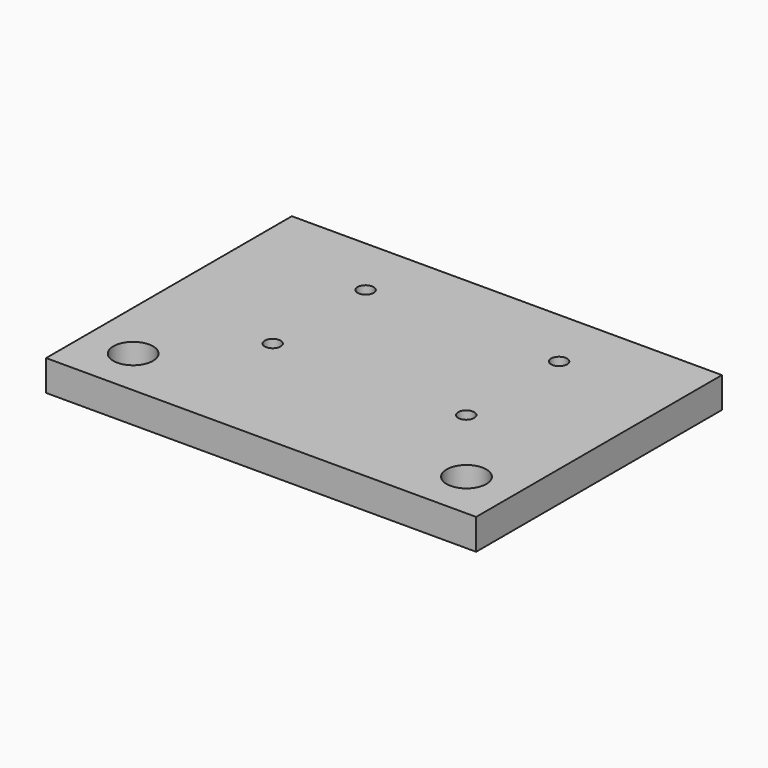
from build123d import *

# Parameters (mm, degrees)
F0_W           = 88.9
F0_H           = 63.5
F1_DEPTH       = 6.35
F2_D           = 8.2042
F3_D           = 3.3
F3_CBORE_D     = 8.25
F3_CBORE_DEPTH = 4


# Not quite as in the source:
# - a feature names something its author has since deleted; it is built from what else it names


with BuildPart() as f1:
    # F0 (on Top) → F1 (new body)
    with BuildSketch(Plane.XY):
        Rectangle(F0_W, F0_H)
    extrude(amount=F1_DEPTH)

    # F2 (through all)
    with Locations(Plane(origin=(0, 0, 0), x_dir=(1, 0, 0), z_dir=(0, 0, -1))):
        with Locations((-34.45, 21.75), (34.45, 21.75)):
            Hole(F2_D / 2)

    # F3 (through all)
    with Locations(Plane(origin=(0, 0, 0), x_dir=(1, 0, 0), z_dir=(0, 0, -1))):
        with Locations((-19.05, -19.05), (-19.05, 4.95), (20.95, -19.05), (20.95, 4.95)):
            CounterBoreHole(F3_D / 2, F3_CBORE_D / 2, F3_CBORE_DEPTH)


solid = f1.part
